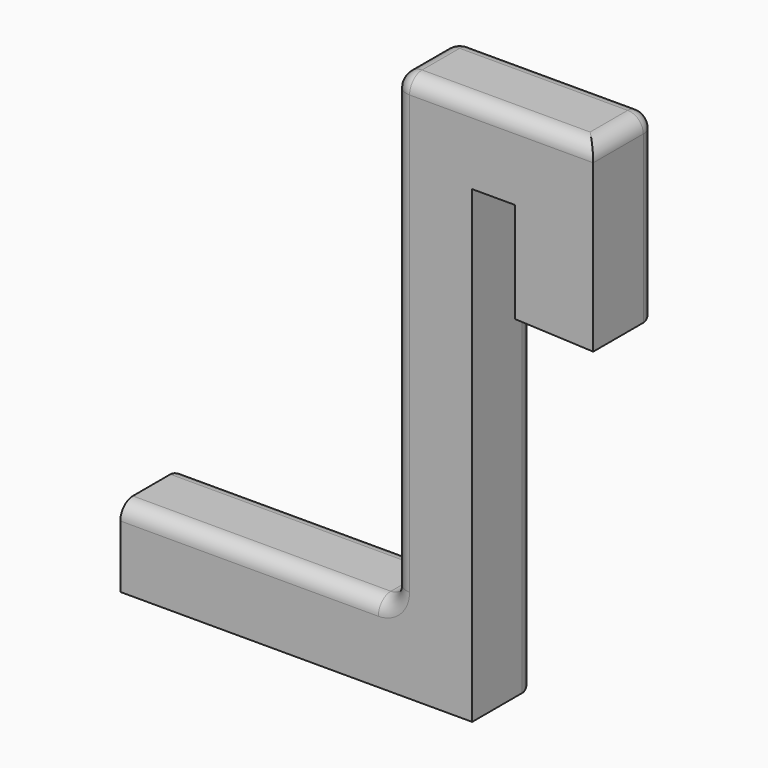
from build123d import *

# Parameters (mm, degrees)
F1_DEPTH     = 25.4
F2_T         = -2.54
F3_T1_DEPTH  = 25.4
F3_S4_W      = 5.08
F3_S4_H      = 5.08
F3_T5_DEPTH  = 5.08
F3_S9_W      = 5.08
F3_S9_H      = 5.08
F3_T10_DEPTH = 5.08
F3_S14_W     = 5.08
F3_S14_H     = 5.08
F3_T15_DEPTH = 5.08
F3_T20_DEPTH = 15.24
F3_T23_DEPTH = 142.24
F3_T26_DEPTH = 142.24
F3_T29_DEPTH = 33.02
F3_T32_DEPTH = 54.5865651855
F3_T35_DEPTH = 72.3665651855
F3_T38_DEPTH = 96.52
F3_T41_DEPTH = 50.8
F3_T44_DEPTH = 139.7
F3_T47_DEPTH = 165.1
F3_T50_DEPTH = 13.9465651855
F3_T53_DEPTH = 45.3396787107
F3_T56_DEPTH = 50.8220888307
F3_T59_DEPTH = 66.7192071509
F3_T62_DEPTH = 96.52
F3_T65_ANGLE = 90
F3_T68_ANGLE = 90
F3_T72_DEPTH = 177.8
F3_T76_DEPTH = 26.6465651855
F3_T82_DEPTH = 26.6465651855
F3_T86_DEPTH = 58.0396787107


# Not quite as in the source:
# - a fillet or chamfer that OpenCascade refuses, or shapes differently, is made with other operations: its cross-section is extruded or revolved along the edge and cut away or added


with BuildPart() as f1:
    # F0 (on Front) → F1 (new body)
    with BuildSketch(Plane.XZ):
        Polygon((-162.270449245, -57.357499212), (-47.970449245, -57.357499212), (-47.970449245, 95.042500788), (-34.0238840595, 95.042500788), (-34.0238840595, 62.4028220773), (-8.6238840595, 61.343293637), (-8.6238840595, 120.442500788), (-73.370449245, 120.442500788), (-73.370449245, 93.7244947603), (-73.370449245, -31.957499212), (-162.270449245, -31.957499212), align=None)
    extrude(amount=F1_DEPTH)

    # F2
    f2_openings = [f1.faces().sort_by_distance(p)[0] for p in [
        (-162.270449, -12.7, -44.657499),
        (-21.323884, -12.7, 61.873058),
    ]]
    offset(amount=F2_T, openings=f2_openings, kind=Kind.INTERSECTION)

    # F3: fillet of radius 5.08 on 16 edges, made by hand

    # F3_s2 → F3_t1 (join)
    with BuildSketch(Plane.XZ):
        with BuildLine():
            ThreePointArc((-78.450449245, -31.957499212), (-74.8583467965, -30.4696016605), (-73.370449245, -26.877499212))
            Line((-73.370449245, -26.877499212), (-73.370449245, -31.957499212))
            Line((-73.370449245, -31.957499212), (-78.450449245, -31.957499212))
        make_face()
    extrude(amount=F3_T1_DEPTH)


with BuildPart() as f3_tool3:
    # F3_s4 → F3_t5 (new body)
    with BuildSketch(Plane.XZ.offset(5.08)):
        with Locations((-70.830449245, 117.902500788)):
            Rectangle(F3_S4_W, F3_S4_H)
    extrude(amount=-F3_T5_DEPTH)

    # F3_s6 → F3_t7 (revolve, cut)
    with BuildSketch(Plane(origin=(-68.290449245, -5.08, 115.362500788), x_dir=(0.7071067812, 0, -0.7071067812), z_dir=(0.7071067812, 0, 0.7071067812))):
        with BuildLine():
            ThreePointArc((0, -5.08), (5.08, 0), (0, 5.08))
            Line((0, 5.08), (0, -5.08))
        make_face()
    revolve(axis=Axis((-68.290449245, -5.08, 115.362500788), (0, 1, 0)), mode=Mode.SUBTRACT)


with BuildPart() as f3_tool8:
    # F3_s9 → F3_t10 (new body)
    with BuildSketch(Plane.XZ.offset(20.32)):
        with Locations((-70.830449245, 117.902500788)):
            Rectangle(F3_S9_W, F3_S9_H)
    extrude(amount=F3_T10_DEPTH)

    # F3_s11 → F3_t12 (revolve, cut)
    with BuildSketch(Plane(origin=(-68.290449245, -20.32, 115.362500788), x_dir=(0.7071067812, 0, -0.7071067812), z_dir=(-0.7071067812, 0, -0.7071067812))):
        with BuildLine():
            ThreePointArc((0, -5.08), (5.08, 0), (0, 5.08))
            Line((0, 5.08), (0, -5.08))
        make_face()
    revolve(axis=Axis((-68.290449245, -20.32, 115.362500788), (0, -1, 0)), mode=Mode.SUBTRACT)


with BuildPart() as f3_tool13:
    # F3_s14 → F3_t15 (new body)
    with BuildSketch(Plane.XZ.offset(5.08)):
        with Locations((-11.1638840595, 117.902500788)):
            Rectangle(F3_S14_W, F3_S14_H)
    extrude(amount=-F3_T15_DEPTH)

    # F3_s16 → F3_t17 (revolve, cut)
    with BuildSketch(Plane(origin=(-13.7038840595, -5.08, 115.362500788), x_dir=(-0.7071067812, 0, -0.7071067812), z_dir=(0.7071067812, 0, -0.7071067812))):
        with BuildLine():
            ThreePointArc((0, -5.08), (5.08, 0), (0, 5.08))
            Line((0, 5.08), (0, -5.08))
        make_face()
    revolve(axis=Axis((-13.7038840595, -5.08, 115.362500788), (0, 1, 0)), mode=Mode.SUBTRACT)


with BuildPart() as f3_tool18:
    # F3_s19 → F3_t20 (new body)
    with BuildSketch(Plane.XZ.offset(5.08)):
        with BuildLine():
            ThreePointArc((-68.290449245, 120.442500788), (-71.8825516934, 118.9546032364), (-73.370449245, 115.362500788))
            Line((-73.370449245, 115.362500788), (-73.370449245, 120.442500788))
            Line((-73.370449245, 120.442500788), (-68.290449245, 120.442500788))
        make_face()
    extrude(amount=F3_T20_DEPTH)


with BuildPart() as f3_tool21:
    # F3_s22 → F3_t23 (new body)
    with BuildSketch(Plane.XY.offset(-26.877499212)):
        with BuildLine():
            ThreePointArc((-68.290449245, -25.4), (-71.8825516934, -23.9121024484), (-73.370449245, -20.32))
            Line((-73.370449245, -20.32), (-73.370449245, -25.4))
            Line((-73.370449245, -25.4), (-68.290449245, -25.4))
        make_face()
    extrude(amount=F3_T23_DEPTH)


with BuildPart() as f3_tool24:
    # F3_s25 → F3_t26 (new body)
    with BuildSketch(Plane.XY.offset(115.362500788)):
        with BuildLine():
            ThreePointArc((-68.290449245, 0), (-71.8825516934, -1.4878975516), (-73.370449245, -5.08))
            Line((-73.370449245, -5.08), (-73.370449245, 0))
            Line((-73.370449245, 0), (-68.290449245, 0))
        make_face()
    extrude(amount=-F3_T26_DEPTH)


with BuildPart() as f3_tool27:
    # F3_s28 → F3_t29 (new body)
    with BuildSketch(Plane.XZ.offset(5.08)):
        with BuildLine():
            ThreePointArc((-8.6238840595, 115.362500788), (-10.1117816111, 118.9546032364), (-13.7038840595, 120.442500788))
            Line((-13.7038840595, 120.442500788), (-8.6238840595, 120.442500788))
            Line((-8.6238840595, 120.442500788), (-8.6238840595, 115.362500788))
        make_face()
    extrude(amount=F3_T29_DEPTH)


with BuildPart() as f3_tool30:
    # F3_s31 → F3_t32 (new body)
    with BuildSketch(Plane.YZ.offset(-13.7038840595)):
        with BuildLine():
            ThreePointArc((0, 115.362500788), (-1.4878975516, 118.9546032364), (-5.08, 120.442500788))
            Line((-5.08, 120.442500788), (0, 120.442500788))
            Line((0, 120.442500788), (0, 115.362500788))
        make_face()
    extrude(amount=-F3_T32_DEPTH)


with BuildPart() as f3_tool33:
    # F3_s34 → F3_t35 (new body)
    with BuildSketch(Plane.YZ.offset(4.0761159405)):
        with BuildLine():
            ThreePointArc((-25.4, 115.362500788), (-23.9121024484, 118.9546032364), (-20.32, 120.442500788))
            Line((-20.32, 120.442500788), (-25.4, 120.442500788))
            Line((-25.4, 120.442500788), (-25.4, 115.362500788))
        make_face()
    extrude(amount=-F3_T35_DEPTH)


with BuildPart() as f3_tool36:
    # F3_s37 → F3_t38 (new body)
    with BuildSketch(Plane.YZ.offset(-78.450449245)):
        with BuildLine():
            ThreePointArc((-5.08, -31.957499212), (-1.4878975516, -33.4453967636), (0, -37.037499212))
            Line((0, -37.037499212), (0, -31.957499212))
            Line((0, -31.957499212), (-5.08, -31.957499212))
        make_face()
    extrude(amount=-F3_T38_DEPTH)


with BuildPart() as f3_tool39:
    # F3_s40 → F3_t41 (new body)
    with BuildSketch(Plane.XY.offset(-19.257499212)):
        with BuildLine():
            ThreePointArc((-157.190449245, 0), (-160.7825516934, -1.4878975516), (-162.270449245, -5.08))
            Line((-162.270449245, -5.08), (-162.270449245, 0))
            Line((-162.270449245, 0), (-157.190449245, 0))
        make_face()
    extrude(amount=-F3_T41_DEPTH)


with BuildPart() as f3_tool42:
    # F3_s43 → F3_t44 (new body)
    with BuildSketch(Plane.YZ.offset(-174.970449245)):
        with BuildLine():
            ThreePointArc((0, -52.277499212), (-1.4878975516, -55.8696016605), (-5.08, -57.357499212))
            Line((-5.08, -57.357499212), (0, -57.357499212))
            Line((0, -57.357499212), (0, -52.277499212))
        make_face()
    extrude(amount=F3_T44_DEPTH)


with BuildPart() as f3_tool45:
    # F3_s46 → F3_t47 (new body)
    with BuildSketch(Plane.XY.offset(-70.057499212)):
        with BuildLine():
            ThreePointArc((-53.050449245, 0), (-49.4583467965, -1.4878975516), (-47.970449245, -5.08))
            Line((-47.970449245, -5.08), (-47.970449245, 0))
            Line((-47.970449245, 0), (-53.050449245, 0))
        make_face()
    extrude(amount=F3_T47_DEPTH)


with BuildPart() as f3_tool48:
    # F3_s49 → F3_t50 (new body)
    with BuildSketch(Plane.YZ.offset(-47.970449245)):
        with BuildLine():
            ThreePointArc((0, 100.122500788), (-1.4878975516, 96.5303983395), (-5.08, 95.042500788))
            Line((-5.08, 95.042500788), (0, 95.042500788))
            Line((0, 95.042500788), (0, 100.122500788))
        make_face()
    extrude(amount=F3_T50_DEPTH)


with BuildPart() as f3_tool51:
    # F3_s52 → F3_t53 (new body)
    with BuildSketch(Plane.XY.offset(95.042500788)):
        with BuildLine():
            ThreePointArc((-28.9438840595, 0), (-32.5359865079, -1.4878975516), (-34.0238840595, -5.08))
            Line((-34.0238840595, -5.08), (-34.0238840595, 0))
            Line((-34.0238840595, 0), (-28.9438840595, 0))
        make_face()
    extrude(amount=-F3_T53_DEPTH)


with BuildPart() as f3_tool54:
    # F3_s55 → F3_t56 (new body)
    with BuildSketch(Plane(origin=(-49.2522815466, 0, 2.0544957892), x_dir=(0, 1, 0), z_dir=(0.9991311166, 0, -0.0416774738))):
        with BuildLine():
            ThreePointArc((0, 66.0105717666), (-1.4878975516, 62.4184693181), (-5.08, 60.9305717666))
            Line((-5.08, 60.9305717666), (0, 60.9305717666))
            Line((0, 60.9305717666), (0, 66.0105717666))
        make_face()
    extrude(amount=F3_T56_DEPTH)


with BuildPart() as f3_tool57:
    # F3_s58 → F3_t59 (new body)
    with BuildSketch(Plane.XY.offset(48.643293637)):
        with BuildLine():
            ThreePointArc((-13.7038840595, 0), (-10.1117816111, -1.4878975516), (-8.6238840595, -5.08))
            Line((-8.6238840595, -5.08), (-8.6238840595, 0))
            Line((-8.6238840595, 0), (-13.7038840595, 0))
        make_face()
    extrude(amount=F3_T59_DEPTH)


with BuildPart() as f3_tool60:
    # F3_s61 → F3_t62 (new body)
    with BuildSketch(Plane.YZ.offset(-78.450449245)):
        with BuildLine():
            ThreePointArc((-20.32, -31.957499212), (-23.9121024484, -33.4453967636), (-25.4, -37.037499212))
            Line((-25.4, -37.037499212), (-25.4, -31.957499212))
            Line((-25.4, -31.957499212), (-20.32, -31.957499212))
        make_face()
    extrude(amount=-F3_T62_DEPTH)


with BuildPart() as f3_tool63:
    # F3_s64 → F3_t65 (revolve)
    with BuildSketch(Plane.YZ.offset(-78.450449245)):
        with BuildLine():
            ThreePointArc((-25.4, -37.037499212), (-23.9121024484, -33.4453967636), (-20.32, -31.957499212))
            Line((-20.32, -31.957499212), (-25.4, -31.957499212))
            Line((-25.4, -31.957499212), (-25.4, -37.037499212))
        make_face()
    revolve(axis=Axis((-78.450449245, -25.4, -26.877499212), (0, -1, 0)), revolution_arc=F3_T65_ANGLE)


with BuildPart() as f3_tool66:
    # F3_s67 → F3_t68 (revolve)
    with BuildSketch(Plane.YZ.offset(-78.450449245)):
        with BuildLine():
            ThreePointArc((0, -37.037499212), (-1.4878975516, -33.4453967636), (-5.08, -31.957499212))
            Line((-5.08, -31.957499212), (0, -31.957499212))
            Line((0, -31.957499212), (0, -37.037499212))
        make_face()
    revolve(axis=Axis((-78.450449245, 0, -26.877499212), (0, -1, 0)), revolution_arc=F3_T68_ANGLE)


with BuildPart() as f3_tool70:
    # F3_s71 → F3_t72 (new body)
    with BuildSketch(Plane.XY.offset(-70.057499212)):
        with BuildLine():
            ThreePointArc((-53.050449245, 0), (-49.4583467965, -1.4878975516), (-47.970449245, -5.08))
            Line((-47.970449245, -5.08), (-47.970449245, 0))
            Line((-47.970449245, 0), (-53.050449245, 0))
        make_face()
    extrude(amount=F3_T72_DEPTH)

    split(bisect_by=Plane.XY.offset(95.042500788), keep=Keep.TOP)


with BuildPart() as f3_tool74:
    # F3_s75 → F3_t76 (new body)
    with BuildSketch(Plane.YZ.offset(-60.670449245)):
        with BuildLine():
            ThreePointArc((0, 100.122500788), (-1.4878975516, 96.5303983395), (-5.08, 95.042500788))
            Line((-5.08, 95.042500788), (0, 95.042500788))
            Line((0, 95.042500788), (0, 100.122500788))
        make_face()
    extrude(amount=F3_T76_DEPTH)

    split(bisect_by=Plane.YZ.offset(-47.970449245), keep=Keep.BOTTOM)


with BuildPart() as f3_tool70_1:
    add(f3_tool70.part)

    # F3_t78: intersect F3_tool74
    add(f3_tool74.part, mode=Mode.INTERSECT)


with BuildPart() as f3_tool80:
    # F3_s81 → F3_t82 (new body)
    with BuildSketch(Plane.YZ.offset(-47.970449245)):
        with BuildLine():
            ThreePointArc((0, 100.122500788), (-1.4878975516, 96.5303983395), (-5.08, 95.042500788))
            Line((-5.08, 95.042500788), (0, 95.042500788))
            Line((0, 95.042500788), (0, 100.122500788))
        make_face()
    extrude(amount=F3_T82_DEPTH)

    split(bisect_by=Plane.YZ.offset(-34.0238840595), keep=Keep.TOP)


with BuildPart() as f3_tool84:
    # F3_s85 → F3_t86 (new body)
    with BuildSketch(Plane.XY.offset(107.742500788)):
        with BuildLine():
            ThreePointArc((-28.9438840595, 0), (-32.5359865079, -1.4878975516), (-34.0238840595, -5.08))
            Line((-34.0238840595, -5.08), (-34.0238840595, 0))
            Line((-34.0238840595, 0), (-28.9438840595, 0))
        make_face()
    extrude(amount=-F3_T86_DEPTH)

    split(bisect_by=Plane.XY.offset(95.042500788), keep=Keep.TOP)


with BuildPart() as f3_tool80_1:
    add(f3_tool80.part)

    # F3_t88: intersect F3_tool84
    add(f3_tool84.part, mode=Mode.INTERSECT)


with BuildPart() as f1_1:
    add(f1.part)

    # F3_t89: cut F3_tool3, F3_tool8, F3_tool13, F3_tool18, F3_tool21, F3_tool24, F3_tool27, F3_tool30, F3_tool33, F3_tool36, F3_tool39, F3_tool42, F3_tool45, F3_tool48, F3_tool51, F3_tool54, F3_tool57, F3_tool60, F3_tool63, F3_tool66, F3_tool70, F3_tool80
    add([f3_tool3.part, f3_tool8.part, f3_tool13.part, f3_tool18.part, f3_tool21.part, f3_tool24.part, f3_tool27.part, f3_tool30.part, f3_tool33.part, f3_tool36.part, f3_tool39.part, f3_tool42.part, f3_tool45.part, f3_tool48.part, f3_tool51.part, f3_tool54.part, f3_tool57.part, f3_tool60.part, f3_tool63.part, f3_tool66.part, f3_tool70_1.part, f3_tool80_1.part], mode=Mode.SUBTRACT)


solid = f1_1.part
